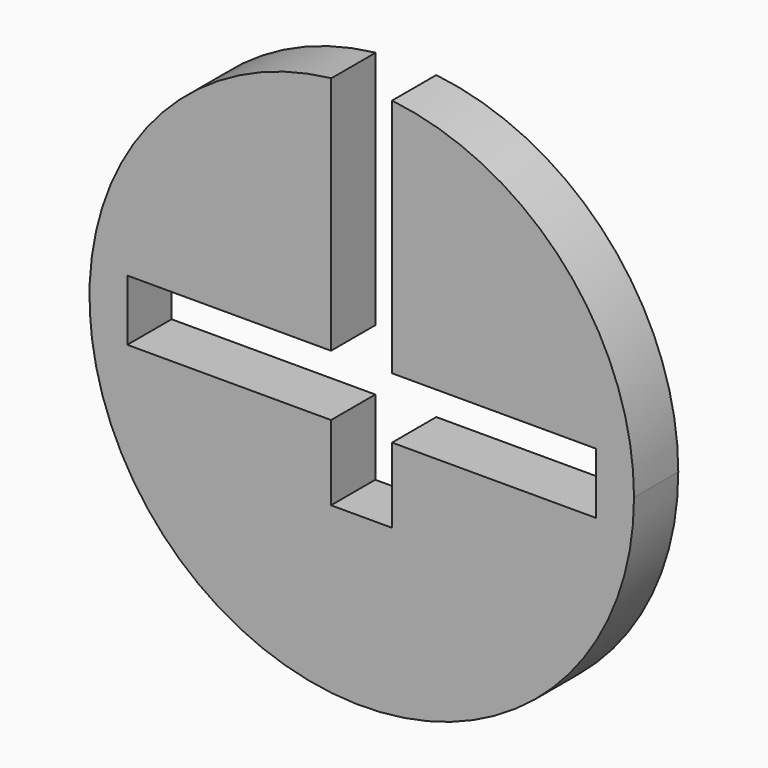
from build123d import *

# Parameters (mm, degrees)
F1_DEPTH = 3.175


# Not quite as in the source:
# - a length typed as a fraction of an inch, garbled in the dataset ("3 / 203.2 mm" for 3/8 in), is restored


with BuildPart() as f1:
    # F0 (on Front) → F1 (new body)
    with BuildSketch(Plane.XZ):
        with BuildLine():
            ThreePointArc((-1.7620097291, 15.5248292089), (-10.4065959669, -11.6545167481), (15.6245, 0))
            ThreePointArc((15.6245, 0), (11.64646361, 10.4156077898), (1.7379902709, 15.52753651))
            Line((1.7379902709, 15.52753651), (1.7379902709, 1.75))
            Line((1.7379902709, 1.75), (13.4525578469, 1.75))
            Line((13.4525578469, 1.75), (13.4525578469, -1.75))
            Line((13.4525578469, -1.75), (1.7379902709, -1.75))
            Line((1.7379902709, -1.75), (1.7379902709, -6.05633948))
            Line((1.7379902709, -6.05633948), (-1.7620097291, -6.05633948))
            Line((-1.7620097291, -6.05633948), (-1.7620097291, -1.75))
            Line((-1.7620097291, -1.75), (-13.4525578469, -1.75))
            Line((-13.4525578469, -1.75), (-13.4525578469, 1.75))
            Line((-13.4525578469, 1.75), (-1.7620097291, 1.75))
            Line((-1.7620097291, 1.75), (-1.7620097291, 15.5248292089))
        make_face()
    extrude(amount=F1_DEPTH)


with BuildPart() as f1b:
    # F0 (on Front) → F1, piece 2 (new body)
    with BuildSketch(Plane.XZ):
        with BuildLine():
            Line((-1.7620097291, 15.52753651), (-1.7620097291, 15.5248292089))
            ThreePointArc((-1.7620097291, 15.5248292089), (-1.7500005235, 15.5261875043), (-1.7379902709, 15.52753651))
            Line((-1.7379902709, 15.52753651), (-1.7620097291, 15.52753651))
        make_face()
    extrude(amount=F1_DEPTH)


solid = Compound([f1.part, f1b.part])
